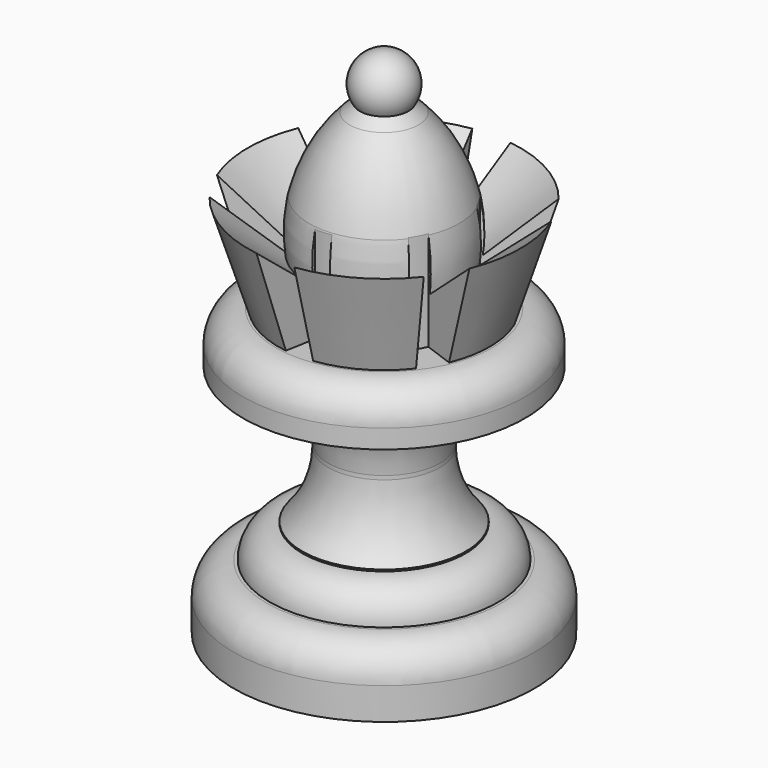
from build123d import *

# Parameters (mm, degrees)
F4_DEPTH = 25


# Not quite as in the source:
# - a feature names something its author has since deleted; it is built from what else it names


with BuildPart() as f1:
    # F0 (on Front) → F1 (revolve)
    with BuildSketch(Plane.XZ):
        with BuildLine():
            Line((-29.0464114308, 0), (0.1370703891, 0))
            Line((0.1370703891, 0), (0.1370703891, 88.2831028199))
            ThreePointArc((0.1370703891, 88.2831028199), (-2.5563679659, 88.9593833587), (-4.6108727149, 90.82779867))
            ThreePointArc((-4.6108727149, 90.82779867), (-5.5976988093, 89.9809104676), (-6.5450577748, 89.0900926644))
            ThreePointArc((-6.5450577748, 89.0900926644), (-11.4568488827, 82.476967596), (-14.4347006416, 74.7963742622))
            ThreePointArc((-14.4347006416, 74.7963742622), (-15.0716593897, 69.8502894666), (-14.8408513427, 64.8687034845))
            Line((-14.8408513427, 64.8687034845), (-26.3505576842, 74.3823973839))
            Line((-26.3505576842, 74.3823973839), (-20.4128239214, 55.6727722287))
            Line((-20.4128239214, 55.6727722287), (-20.9242871106, 55.6727722287))
            ThreePointArc((-20.9242871106, 55.6727722287), (-25.4144151711, 53.8129002893), (-27.2742871106, 49.3227722287))
            Line((-27.2742871106, 49.3227722287), (-27.2742871106, 45.666474849))
            Line((-27.2742871106, 45.666474849), (-15.7439641526, 45.666474849))
            Line((-15.7439641526, 45.666474849), (-15.7439641526, 45.3329899947))
            ThreePointArc((-15.7439641526, 45.3329899947), (-12.1015621728, 39.422032357), (-10.7439633369, 32.612962099))
            ThreePointArc((-10.7439633369, 32.612962099), (-10.7403918284, 32.2384637675), (-10.7439633369, 31.863965436))
            ThreePointArc((-10.7439633369, 31.863965436), (-12.1015621728, 25.054895178), (-15.7439641526, 19.1439375403))
            Line((-15.7439641526, 19.1439375403), (-15.7439641526, 18.810452686))
            ThreePointArc((-15.7439641526, 18.810452686), (-20.2340922131, 16.9505807466), (-22.0939641526, 12.460452686))
            Line((-22.0939641526, 12.460452686), (-22.0939641526, 12.5479437411))
            Line((-22.0939641526, 12.5479437411), (-22.6964114308, 12.5479437411))
            ThreePointArc((-22.6964114308, 12.5479437411), (-27.1865394914, 10.6880718016), (-29.0464114308, 6.1979437411))
            Line((-29.0464114308, 6.1979437411), (-29.0464114308, 0))
        make_face()
        with BuildLine():
            ThreePointArc((-4.6108727149, 90.82779867), (-2.5563679659, 88.9593833587), (0.1370703891, 88.2831028199))
            Line((0.1370703891, 88.2831028199), (0.1370703891, 93.9848531267))
            Line((0.1370703891, 93.9848531267), (0.1370703891, 99.6866034335))
            ThreePointArc((0.1370703891, 99.6866034335), (-4.8883993789, 96.6782914817), (-4.6108727149, 90.82779867))
        make_face()
        with BuildLine():
            Line((-10.7439633369, 32.612962099), (-10.7439633369, 31.863965436))
            ThreePointArc((-10.7439633369, 31.863965436), (-10.7403918284, 32.2384637675), (-10.7439633369, 32.612962099))
        make_face()
    revolve(axis=Axis((0.1370703891, 0, 46.9924265633), (0, 0, -1)))

    # F3 (on face) → F4 (cut)
    with BuildSketch(Plane.XY.offset(55.6727722287)):
        with BuildLine():
            ThreePointArc((-1.6347205774, 14.5514276956), (0, 14.6429627926), (1.6347205774, 14.5514276956))
            Line((1.6347205774, 14.5514276956), (4.9368817802, 33.2789144903))
            ThreePointArc((4.9368817802, 33.2789144903), (0, 33.6431114995), (-4.9368817802, 33.2789144903))
            Line((-4.9368817802, 33.2789144903), (-1.6347205774, 14.5514276956))
        make_face()
        with BuildLine():
            ThreePointArc((-13.4192663344, 5.8600042997), (-12.681177765, 7.3214813963), (-11.784545757, 8.6914233959))
            Line((-11.784545757, 8.6914233959), (-26.3519444689, 20.9149222823))
            ThreePointArc((-26.3519444689, 20.9149222823), (-29.1357892209, 16.8215557497), (-31.2888262491, 12.3639922081))
            Line((-31.2888262491, 12.3639922081), (-13.4192663344, 5.8600042997))
        make_face()
        with BuildLine():
            ThreePointArc((-11.784545757, -8.6914233959), (-12.681177765, -7.3214813963), (-13.4192663344, -5.8600042997))
            Line((-13.4192663344, -5.8600042997), (-31.2888262491, -12.3639922081))
            ThreePointArc((-31.2888262491, -12.3639922081), (-29.1357892209, -16.8215557497), (-26.3519444689, -20.9149222823))
            Line((-26.3519444689, -20.9149222823), (-11.784545757, -8.6914233959))
        make_face()
        with BuildLine():
            ThreePointArc((1.6347205774, -14.5514276956), (0, -14.6429627926), (-1.6347205774, -14.5514276956))
            Line((-1.6347205774, -14.5514276956), (-4.9368817802, -33.2789144903))
            ThreePointArc((-4.9368817802, -33.2789144903), (0, -33.6431114995), (4.9368817802, -33.2789144903))
            Line((4.9368817802, -33.2789144903), (1.6347205774, -14.5514276956))
        make_face()
        with BuildLine():
            ThreePointArc((13.4192663344, -5.8600042997), (12.681177765, -7.3214813963), (11.784545757, -8.6914233959))
            Line((11.784545757, -8.6914233959), (26.3519444689, -20.9149222823))
            ThreePointArc((26.3519444689, -20.9149222823), (29.1357892209, -16.8215557497), (31.2888262491, -12.3639922081))
            Line((31.2888262491, -12.3639922081), (13.4192663344, -5.8600042997))
        make_face()
        with BuildLine():
            ThreePointArc((11.784545757, 8.6914233959), (12.681177765, 7.3214813963), (13.4192663344, 5.8600042997))
            Line((13.4192663344, 5.8600042997), (31.2888262491, 12.3639922081))
            ThreePointArc((31.2888262491, 12.3639922081), (29.1357892209, 16.8215557497), (26.3519444689, 20.9149222823))
            Line((26.3519444689, 20.9149222823), (11.784545757, 8.6914233959))
        make_face()
    extrude(amount=F4_DEPTH, mode=Mode.SUBTRACT)


solid = f1.part
